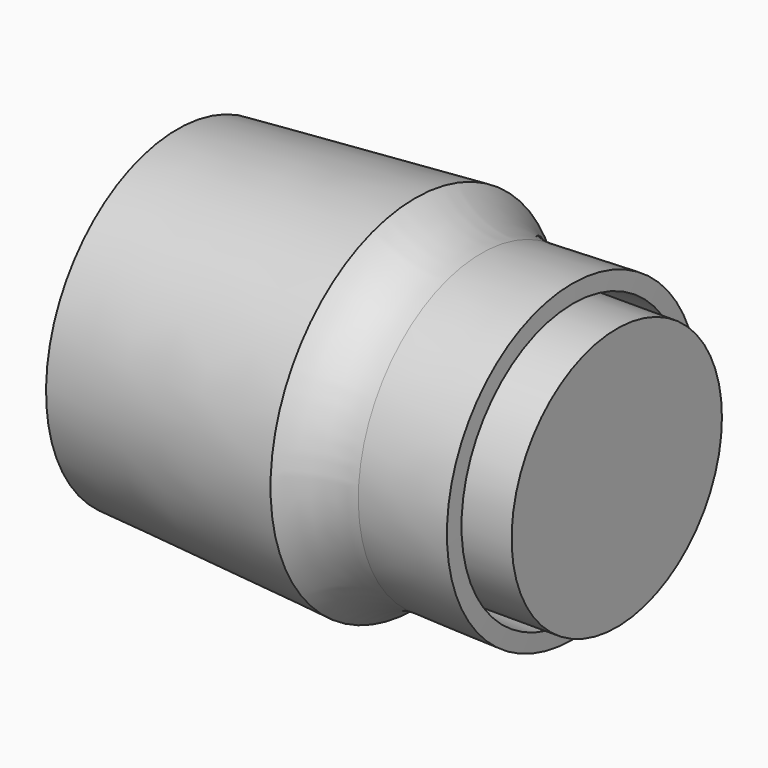
from build123d import *

# Parameters (mm, degrees)
F1_R     = 15
F2_DEPTH = 25


# Not quite as in the source:
# - a fillet or chamfer that OpenCascade refuses, or shapes differently, is made with other operations: its cross-section is extruded or revolved along the edge and cut away or added


with BuildPart() as f2:
    # F1 (on Right) → F2 (new body)
    with BuildSketch(Plane.YZ):
        Circle(F1_R)
    extrude(amount=F2_DEPTH)


with BuildPart() as f3:
    # F3: sweep along a path in F3_path
    with BuildLine(Plane(origin=(0, 15, 0), x_dir=(0, 0, -1), z_dir=(-1, 0, 0))) as f3_path:
        CenterArc((0, 15), 15, 0, 360)
    # F0 (on Front) → F3 (sweep)
    with BuildSketch(Plane.XZ):
        Polygon((0, 18.5), (0, 15.25), (20, 15.9), (19.935034301, 17.898944586), (2, 17.3160559712), (2, 20.6448940122), (-25.1396582554, 18.7451179343), (-25, 16.75), align=None)
    sweep(path=f3_path.line)

    # F4: fillet of radius 10 on 1 edges, made by hand

    # F4_s1 → F4_t2 (revolve)
    with BuildSketch(Plane.XZ):
        with BuildLine():
            ThreePointArc((9.5521060353, -17.5614994174), (5.4473593848, -18.2981329798), (2, -20.6448940122))
            Line((2, -20.6448940122), (1.8554544492, -20.5066674455))
            ThreePointArc((1.8554544492, -20.5066674455), (1.8, -18.9804749917), (1.8, -17.3160559712))
            Line((1.8, -17.3160559712), (2.0064965699, -17.1161615126))
            Line((2.0064965699, -17.1161615126), (9.5586026053, -17.3616049588))
            Line((9.5586026053, -17.3616049588), (9.5521060353, -17.5614994174))
        make_face()
    revolve(axis=Axis((2, 0, 0), (-1, 0, 0)))


solid = Compound([f2.part, f3.part])
